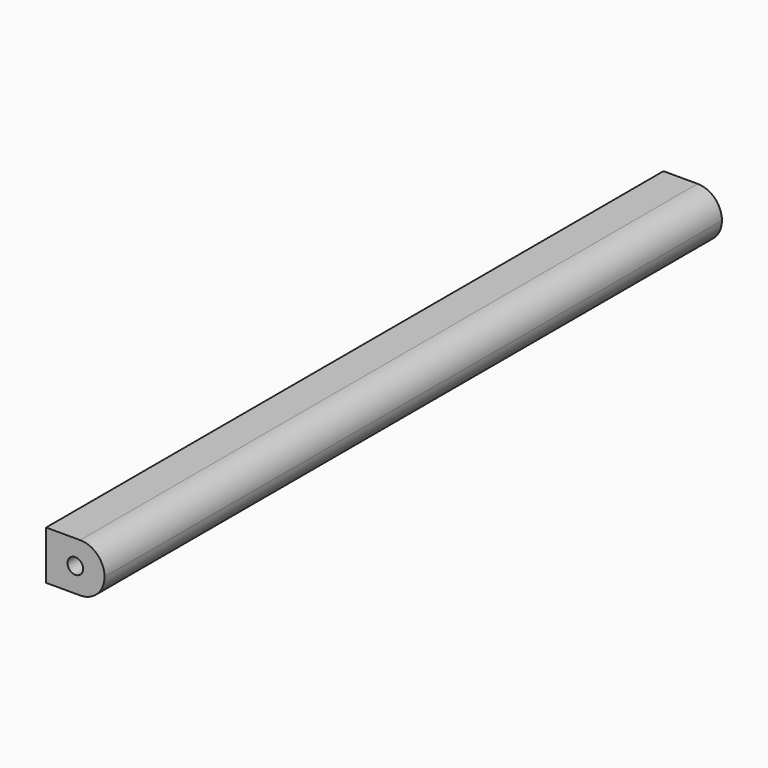
from build123d import *

# Parameters (mm, degrees)
F1_DEPTH = 7.62
F2_R     = 3.17499
F4_R     = 1.016
F5_DEPTH = 7.62
F3_R     = 1.016
F6_DEPTH = 7.62


# Not quite as in the source:
# - a fillet or chamfer is up to 0.001 mm smaller than in the source, because OpenCascade refuses the exact size


with BuildPart() as f1:
    # F0 (on Right) → F1 (new body)
    with BuildSketch(Plane.YZ):
        Polygon((50.292, -3.175), (50.292, 3.175), (0, 3.175), (-50.292, 3.175), (-50.292, -3.175), align=None)
    extrude(amount=F1_DEPTH)

    # F2 (radius 3.175 in the source; OpenCascade refuses exactly that, so slightly less here)
    f2_edges = [f1.edges().sort_by_distance(p)[0] for p in [
        (7.62, 0, -3.175),
        (7.62, 0, 3.175),
    ]]
    fillet(f2_edges, radius=F2_R)

    # F4 (on face) → F5 (cut)
    with BuildSketch(Plane.XZ.offset(50.292)):
        with Locations((3.81, 0)):
            Circle(F4_R)
    extrude(amount=-F5_DEPTH, mode=Mode.SUBTRACT)

    # F3 (on face) → F6 (cut)
    with BuildSketch(Plane(origin=(0, 50.292, 0), x_dir=(-1, 0, 0), z_dir=(0, 1, 0))):
        with Locations((-3.81, 0)):
            Circle(F3_R)
    extrude(amount=-F6_DEPTH, mode=Mode.SUBTRACT)


solid = f1.part
